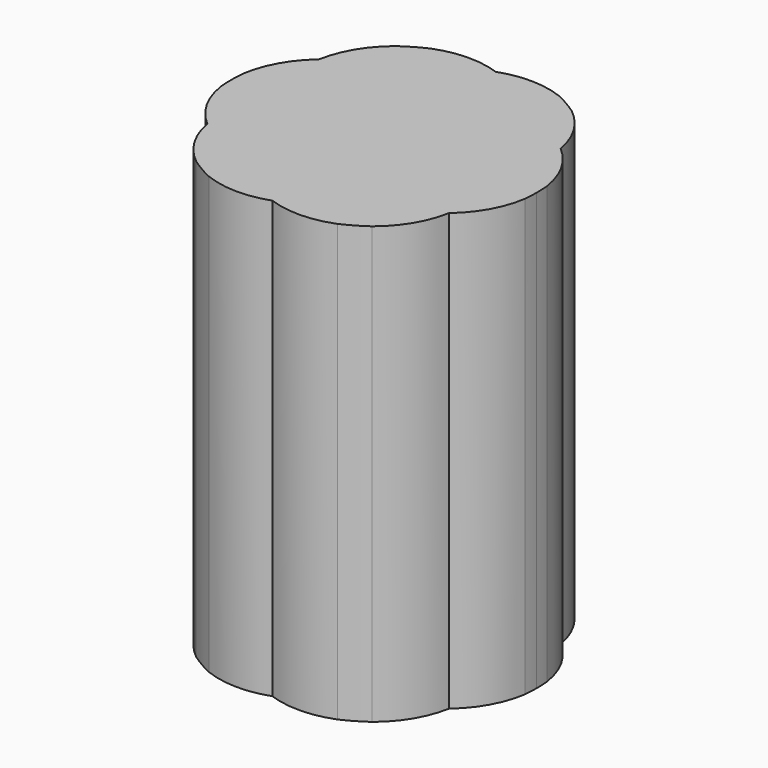
from build123d import *

# Parameters (mm, degrees)
F1_DEPTH = 5


with BuildPart() as f1:
    # F0 (on Top) → F1 (new body)
    with BuildSketch(Plane.XY):
        with BuildLine():
            ThreePointArc((1.7429623373, -0.1567874062), (1.748239699, -0.0784726376), (1.75, 0))
            ThreePointArc((1.75, 0), (1.748239699, 0.0784726376), (1.7429623373, 0.1567874062))
            ThreePointArc((1.7429623373, 0.1567874062), (1.6222133761, 0.5106191558), (1.3851445143, 0.7997135582))
            ThreePointArc((1.3851445143, 0.7997135582), (1.3980525813, 0.7054063545), (1.4023670894, 0.6103177017))
            ThreePointArc((1.4023670894, 0.6103177017), (1.3522740733, 0.2898711016), (1.2067746637, 0))
            ThreePointArc((1.2067746637, 0), (1.3522740733, -0.2898711016), (1.4023670894, -0.6103177017))
            ThreePointArc((1.4023670894, -0.6103177017), (1.3980525813, -0.7054063545), (1.3851445143, -0.7997135582))
            ThreePointArc((1.3851445143, -0.7997135582), (1.6222133761, -0.5106191558), (1.7429623373, -0.1567874062))
        make_face()
        with BuildLine():
            ThreePointArc((1.3851445143, 0.7997135582), (1.2533158487, 1.1495684162), (1.0072630454, 1.4310559589))
            ThreePointArc((1.0072630454, 1.4310559589), (0.875, 1.5155444566), (0.7356992919, 1.587843365))
            ThreePointArc((0.7356992919, 1.587843365), (0.3688975274, 1.660187572), (0, 1.5994271164))
            ThreePointArc((0, 1.5994271164), (0.357996056, 1.3835474229), (0.6033873318, 1.0450975154))
            ThreePointArc((0.6033873318, 1.0450975154), (1.0191891876, 1.0018073904), (1.3851445143, 0.7997135582))
        make_face()
        with BuildLine():
            ThreePointArc((1.4023670894, 0.6103177017), (1.3980525813, 0.7054063545), (1.3851445143, 0.7997135582))
            ThreePointArc((1.3851445143, 0.7997135582), (1.0191891876, 1.0018073904), (0.6033873318, 1.0450975154))
            ThreePointArc((0.6033873318, 1.0450975154), (0.6738010602, 0.8327562974), (0.6976329106, 0.6103177017))
            ThreePointArc((0.6976329106, 0.6103177017), (0.6917287242, 0.4991244824), (0.6740825639, 0.3891817497))
            ThreePointArc((0.6740825639, 0.3891817497), (0.9717877583, 0.23751367), (1.2067746637, 0))
            ThreePointArc((1.2067746637, 0), (1.3522740733, 0.2898711016), (1.4023670894, 0.6103177017))
        make_face()
        with BuildLine():
            ThreePointArc((0.7356992919, -1.587843365), (0.875, -1.5155444566), (1.0072630454, -1.4310559589))
            ThreePointArc((1.0072630454, -1.4310559589), (1.2533158487, -1.1495684162), (1.3851445143, -0.7997135582))
            ThreePointArc((1.3851445143, -0.7997135582), (1.0191891876, -1.0018073904), (0.6033873318, -1.0450975154))
            ThreePointArc((0.6033873318, -1.0450975154), (0.357996056, -1.3835474229), (0, -1.5994271164))
            ThreePointArc((0, -1.5994271164), (0.3688975274, -1.660187572), (0.7356992919, -1.587843365))
        make_face()
        with BuildLine():
            ThreePointArc((0.6033873318, -1.0450975154), (1.0191891876, -1.0018073904), (1.3851445143, -0.7997135582))
            ThreePointArc((1.3851445143, -0.7997135582), (1.3980525813, -0.7054063545), (1.4023670894, -0.6103177017))
            ThreePointArc((1.4023670894, -0.6103177017), (1.3522740733, -0.2898711016), (1.2067746637, 0))
            ThreePointArc((1.2067746637, 0), (0.9717877583, -0.23751367), (0.6740825639, -0.3891817497))
            ThreePointArc((0.6740825639, -0.3891817497), (0.6917287242, -0.4991244824), (0.6976329106, -0.6103177017))
            ThreePointArc((0.6976329106, -0.6103177017), (0.6738010602, -0.8327562974), (0.6033873318, -1.0450975154))
        make_face()
        with BuildLine():
            ThreePointArc((0.6976329106, 0.6103177017), (0.6738010602, 0.8327562974), (0.6033873318, 1.0450975154))
            ThreePointArc((0.6033873318, 1.0450975154), (0.2802010071, 0.9603497208), (0, 0.7783634995))
            ThreePointArc((0, 0.7783634995), (0.143097193, 0.6194206689), (0.2510202425, 0.4347798137))
            ThreePointArc((0.2510202425, 0.4347798137), (0.4648854384, 0.4336361388), (0.6740825639, 0.3891817497))
            ThreePointArc((0.6740825639, 0.3891817497), (0.6917287242, 0.4991244824), (0.6976329106, 0.6103177017))
        make_face()
        with BuildLine():
            ThreePointArc((0, 0.7783634995), (0.2802010071, 0.9603497208), (0.6033873318, 1.0450975154))
            ThreePointArc((0.6033873318, 1.0450975154), (0.357996056, 1.3835474229), (0, 1.5994271164))
            ThreePointArc((0, 1.5994271164), (-0.357996056, 1.3835474229), (-0.6033873318, 1.0450975154))
            ThreePointArc((-0.6033873318, 1.0450975154), (-0.2802010071, 0.9603497208), (0, 0.7783634995))
        make_face()
        with BuildLine():
            ThreePointArc((0, -0.7783634995), (0.2802010071, -0.9603497208), (0.6033873318, -1.0450975154))
            ThreePointArc((0.6033873318, -1.0450975154), (0.6738010602, -0.8327562974), (0.6976329106, -0.6103177017))
            ThreePointArc((0.6976329106, -0.6103177017), (0.6917287242, -0.4991244824), (0.6740825639, -0.3891817497))
            ThreePointArc((0.6740825639, -0.3891817497), (0.4648854384, -0.4336361388), (0.2510202425, -0.4347798137))
            ThreePointArc((0.2510202425, -0.4347798137), (0.143097193, -0.6194206689), (0, -0.7783634995))
        make_face()
        with BuildLine():
            ThreePointArc((0, -1.5994271164), (0.357996056, -1.3835474229), (0.6033873318, -1.0450975154))
            ThreePointArc((0.6033873318, -1.0450975154), (0.2802010071, -0.9603497208), (0, -0.7783634995))
            ThreePointArc((0, -0.7783634995), (-0.2802010071, -0.9603497208), (-0.6033873318, -1.0450975154))
            ThreePointArc((-0.6033873318, -1.0450975154), (-0.357996056, -1.3835474229), (0, -1.5994271164))
        make_face()
        with BuildLine():
            ThreePointArc((0, 1.5994271164), (-0.3688975274, 1.660187572), (-0.7356992919, 1.587843365))
            ThreePointArc((-0.7356992919, 1.587843365), (-0.875, 1.5155444566), (-1.0072630454, 1.4310559589))
            ThreePointArc((-1.0072630454, 1.4310559589), (-1.2533158487, 1.1495684162), (-1.3851445143, 0.7997135582))
            ThreePointArc((-1.3851445143, 0.7997135582), (-1.0191891876, 1.0018073904), (-0.6033873318, 1.0450975154))
            ThreePointArc((-0.6033873318, 1.0450975154), (-0.357996056, 1.3835474229), (0, 1.5994271164))
        make_face()
        with BuildLine():
            ThreePointArc((-0.2510202425, 0.4347798137), (-0.143097193, 0.6194206689), (0, 0.7783634995))
            ThreePointArc((0, 0.7783634995), (-0.2802010071, 0.9603497208), (-0.6033873318, 1.0450975154))
            ThreePointArc((-0.6033873318, 1.0450975154), (-0.6915867512, 0.7228360507), (-0.6740825639, 0.3891817497))
            ThreePointArc((-0.6740825639, 0.3891817497), (-0.4648854384, 0.4336361388), (-0.2510202425, 0.4347798137))
        make_face()
        with BuildLine():
            ThreePointArc((0.2510202425, 0.4347798137), (0.143097193, 0.6194206689), (0, 0.7783634995))
            ThreePointArc((0, 0.7783634995), (-0.143097193, 0.6194206689), (-0.2510202425, 0.4347798137))
            ThreePointArc((-0.2510202425, 0.4347798137), (-0.1237894202, 0.4145004525), (0, 0.3787917131))
            ThreePointArc((0, 0.3787917131), (0.1237894202, 0.4145004525), (0.2510202425, 0.4347798137))
        make_face()
        with BuildLine():
            ThreePointArc((0.6740825639, -0.3891817497), (0.9717877583, -0.23751367), (1.2067746637, 0))
            ThreePointArc((1.2067746637, 0), (0.9717877583, 0.23751367), (0.6740825639, 0.3891817497))
            ThreePointArc((0.6740825639, 0.3891817497), (0.6079826314, 0.1857845301), (0.5020404849, 0))
            ThreePointArc((0.5020404849, 0), (0.6079826314, -0.1857845301), (0.6740825639, -0.3891817497))
        make_face()
        with BuildLine():
            ThreePointArc((-1.0072630454, -1.4310559589), (-0.875, -1.5155444566), (-0.7356992919, -1.587843365))
            ThreePointArc((-0.7356992919, -1.587843365), (-0.3688975274, -1.660187572), (0, -1.5994271164))
            ThreePointArc((0, -1.5994271164), (-0.357996056, -1.3835474229), (-0.6033873318, -1.0450975154))
            ThreePointArc((-0.6033873318, -1.0450975154), (-1.0191891876, -1.0018073904), (-1.3851445143, -0.7997135582))
            ThreePointArc((-1.3851445143, -0.7997135582), (-1.2533158487, -1.1495684162), (-1.0072630454, -1.4310559589))
        make_face()
        with BuildLine():
            ThreePointArc((-0.2510202425, -0.4347798137), (-0.143097193, -0.6194206689), (0, -0.7783634995))
            ThreePointArc((0, -0.7783634995), (0.143097193, -0.6194206689), (0.2510202425, -0.4347798137))
            ThreePointArc((0.2510202425, -0.4347798137), (0.1237894202, -0.4145004525), (0, -0.3787917131))
            ThreePointArc((0, -0.3787917131), (-0.1237894202, -0.4145004525), (-0.2510202425, -0.4347798137))
        make_face()
        with BuildLine():
            ThreePointArc((-0.6033873318, -1.0450975154), (-0.2802010071, -0.9603497208), (0, -0.7783634995))
            ThreePointArc((0, -0.7783634995), (-0.143097193, -0.6194206689), (-0.2510202425, -0.4347798137))
            ThreePointArc((-0.2510202425, -0.4347798137), (-0.4648854384, -0.4336361388), (-0.6740825639, -0.3891817497))
            ThreePointArc((-0.6740825639, -0.3891817497), (-0.6915867512, -0.7228360507), (-0.6033873318, -1.0450975154))
        make_face()
        with BuildLine():
            ThreePointArc((-0.6740825639, 0.3891817497), (-0.6915867512, 0.7228360507), (-0.6033873318, 1.0450975154))
            ThreePointArc((-0.6033873318, 1.0450975154), (-1.0191891876, 1.0018073904), (-1.3851445143, 0.7997135582))
            ThreePointArc((-1.3851445143, 0.7997135582), (-1.3771852436, 0.3817400325), (-1.2067746637, 0))
            ThreePointArc((-1.2067746637, 0), (-0.9717877583, 0.23751367), (-0.6740825639, 0.3891817497))
        make_face()
        with BuildLine():
            ThreePointArc((0.6740825639, 0.3891817497), (0.4648854384, 0.4336361388), (0.2510202425, 0.4347798137))
            ThreePointArc((0.2510202425, 0.4347798137), (0.2970732116, 0.3144550089), (0.3280432462, 0.1893958565))
            ThreePointArc((0.3280432462, 0.1893958565), (0.4208626318, 0.1000454436), (0.5020404849, 0))
            ThreePointArc((0.5020404849, 0), (0.6079826314, 0.1857845301), (0.6740825639, 0.3891817497))
        make_face()
        with BuildLine():
            ThreePointArc((0.3280432462, 0.1893958565), (0.2970732116, 0.3144550089), (0.2510202425, 0.4347798137))
            ThreePointArc((0.2510202425, 0.4347798137), (0.1237894202, 0.4145004525), (0, 0.3787917131))
            ThreePointArc((0, 0.3787917131), (0.1726329106, 0.2990089723), (0.3280432462, 0.1893958565))
        make_face()
        with BuildLine():
            ThreePointArc((-0.3280432462, 0.1893958565), (-0.2970732116, 0.3144550089), (-0.2510202425, 0.4347798137))
            ThreePointArc((-0.2510202425, 0.4347798137), (-0.4648854384, 0.4336361388), (-0.6740825639, 0.3891817497))
            ThreePointArc((-0.6740825639, 0.3891817497), (-0.6079826314, 0.1857845301), (-0.5020404849, 0))
            ThreePointArc((-0.5020404849, 0), (-0.4208626318, 0.1000454436), (-0.3280432462, 0.1893958565))
        make_face()
        with BuildLine():
            ThreePointArc((0, 0.3787917131), (-0.1237894202, 0.4145004525), (-0.2510202425, 0.4347798137))
            ThreePointArc((-0.2510202425, 0.4347798137), (-0.2970732116, 0.3144550089), (-0.3280432462, 0.1893958565))
            ThreePointArc((-0.3280432462, 0.1893958565), (-0.1726329106, 0.2990089723), (0, 0.3787917131))
        make_face()
        with BuildLine():
            ThreePointArc((0.2510202425, -0.4347798137), (0.4648854384, -0.4336361388), (0.6740825639, -0.3891817497))
            ThreePointArc((0.6740825639, -0.3891817497), (0.6079826314, -0.1857845301), (0.5020404849, 0))
            ThreePointArc((0.5020404849, 0), (0.4208626318, -0.1000454436), (0.3280432462, -0.1893958565))
            ThreePointArc((0.3280432462, -0.1893958565), (0.2970732116, -0.3144550089), (0.2510202425, -0.4347798137))
        make_face()
        with BuildLine():
            ThreePointArc((-1.3851445143, -0.7997135582), (-1.0191891876, -1.0018073904), (-0.6033873318, -1.0450975154))
            ThreePointArc((-0.6033873318, -1.0450975154), (-0.6915867512, -0.7228360507), (-0.6740825639, -0.3891817497))
            ThreePointArc((-0.6740825639, -0.3891817497), (-0.9717877583, -0.23751367), (-1.2067746637, 0))
            ThreePointArc((-1.2067746637, 0), (-1.3771852436, -0.3817400325), (-1.3851445143, -0.7997135582))
        make_face()
        with BuildLine():
            ThreePointArc((0, -0.3787917131), (0.1237894202, -0.4145004525), (0.2510202425, -0.4347798137))
            ThreePointArc((0.2510202425, -0.4347798137), (0.2970732116, -0.3144550089), (0.3280432462, -0.1893958565))
            ThreePointArc((0.3280432462, -0.1893958565), (0.1726329106, -0.2990089723), (0, -0.3787917131))
        make_face()
        with BuildLine():
            ThreePointArc((-0.6740825639, -0.3891817497), (-0.4648854384, -0.4336361388), (-0.2510202425, -0.4347798137))
            ThreePointArc((-0.2510202425, -0.4347798137), (-0.2970732116, -0.3144550089), (-0.3280432462, -0.1893958565))
            ThreePointArc((-0.3280432462, -0.1893958565), (-0.4208626318, -0.1000454436), (-0.5020404849, 0))
            ThreePointArc((-0.5020404849, 0), (-0.6079826314, -0.1857845301), (-0.6740825639, -0.3891817497))
        make_face()
        with BuildLine():
            ThreePointArc((-0.3280432462, -0.1893958565), (-0.2970732116, -0.3144550089), (-0.2510202425, -0.4347798137))
            ThreePointArc((-0.2510202425, -0.4347798137), (-0.1237894202, -0.4145004525), (0, -0.3787917131))
            ThreePointArc((0, -0.3787917131), (-0.1726329106, -0.2990089723), (-0.3280432462, -0.1893958565))
        make_face()
        with BuildLine():
            ThreePointArc((-1.3851445143, 0.7997135582), (-1.6222133761, 0.5106191558), (-1.7429623373, 0.1567874062))
            ThreePointArc((-1.7429623373, 0.1567874062), (-1.75, 0), (-1.7429623373, -0.1567874062))
            ThreePointArc((-1.7429623373, -0.1567874062), (-1.6222133761, -0.5106191558), (-1.3851445143, -0.7997135582))
            ThreePointArc((-1.3851445143, -0.7997135582), (-1.3771852436, -0.3817400325), (-1.2067746637, 0))
            ThreePointArc((-1.2067746637, 0), (-1.3771852436, 0.3817400325), (-1.3851445143, 0.7997135582))
        make_face()
        with BuildLine():
            ThreePointArc((-0.5020404849, 0), (-0.6079826314, 0.1857845301), (-0.6740825639, 0.3891817497))
            ThreePointArc((-0.6740825639, 0.3891817497), (-0.9717877583, 0.23751367), (-1.2067746637, 0))
            ThreePointArc((-1.2067746637, 0), (-0.9717877583, -0.23751367), (-0.6740825639, -0.3891817497))
            ThreePointArc((-0.6740825639, -0.3891817497), (-0.6079826314, -0.1857845301), (-0.5020404849, 0))
        make_face()
        with BuildLine():
            ThreePointArc((0.5020404849, 0), (0.4208626318, 0.1000454436), (0.3280432462, 0.1893958565))
            ThreePointArc((0.3280432462, 0.1893958565), (0.3409513132, 0.0950886528), (0.3452658213, 0))
            ThreePointArc((0.3452658213, 0), (0.3409513132, -0.0950886528), (0.3280432462, -0.1893958565))
            ThreePointArc((0.3280432462, -0.1893958565), (0.4208626318, -0.1000454436), (0.5020404849, 0))
        make_face()
        with BuildLine():
            ThreePointArc((0.3452658213, 0), (0.3409513132, 0.0950886528), (0.3280432462, 0.1893958565))
            ThreePointArc((0.3280432462, 0.1893958565), (0.1726329106, 0.2990089723), (0, 0.3787917131))
            ThreePointArc((0, 0.3787917131), (-0.1726329106, 0.2990089723), (-0.3280432462, 0.1893958565))
            ThreePointArc((-0.3280432462, 0.1893958565), (-0.3452658213, 0), (-0.3280432462, -0.1893958565))
            ThreePointArc((-0.3280432462, -0.1893958565), (-0.1726329106, -0.2990089723), (0, -0.3787917131))
            ThreePointArc((0, -0.3787917131), (0.1726329106, -0.2990089723), (0.3280432462, -0.1893958565))
            ThreePointArc((0.3280432462, -0.1893958565), (0.3409513132, -0.0950886528), (0.3452658213, 0))
        make_face()
        with BuildLine():
            ThreePointArc((-0.3280432462, -0.1893958565), (-0.3452658213, 0), (-0.3280432462, 0.1893958565))
            ThreePointArc((-0.3280432462, 0.1893958565), (-0.4208626318, 0.1000454436), (-0.5020404849, 0))
            ThreePointArc((-0.5020404849, 0), (-0.4208626318, -0.1000454436), (-0.3280432462, -0.1893958565))
        make_face()
    extrude(amount=F1_DEPTH)


solid = f1.part
